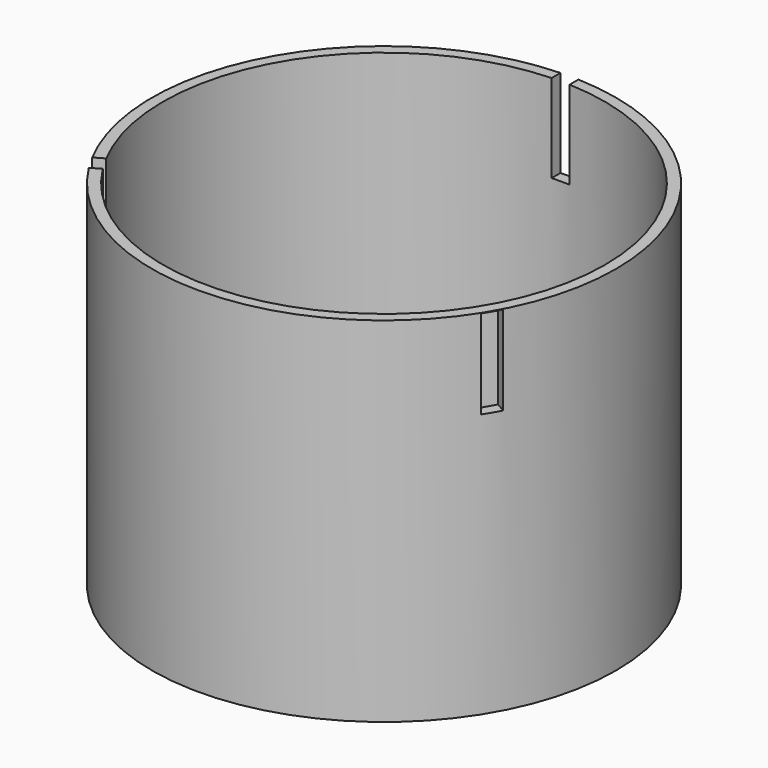
from build123d import *

# Parameters (mm, degrees)
F0_R           = 33.3375
F1_DEPTH       = 50.8
F2_T           = -1.5875
F6_W           = 2.5429241359
F6_H           = 13.1887868047
F7_DEPTH       = 12.7
F10_W          = 2.6744855568
F10_H          = 12.775093317
F11_DEPTH      = 2.794
F11_DEPTH_BACK = 2.413
F13_W          = 2.5820170995
F13_H          = 12.7615630627
F14_DEPTH      = 5.0546
F14_DEPTH_BACK = 4.7244
F15_W          = 7.62
F15_H          = 31.75
F15_R          = 1.397
F16_DEPTH      = 9.906


# Not quite as in the source:
# - a feature names something its author has since deleted; it is built from what else it names


with BuildPart() as f1:
    # F0 (on Top) → F1 (new body)
    with BuildSketch(Plane.XY):
        Circle(F0_R)
    extrude(amount=F1_DEPTH)

    # F2
    f2_openings = [f1.faces().sort_by_distance(p)[0] for p in [
        (0, 0, 50.8),
    ]]
    offset(amount=F2_T, openings=f2_openings)

    # F6 (on offset) → F7 (cut)
    with BuildSketch(Plane(origin=(-28.8711218987, -16.66875, 0), x_dir=(0.5, -0.8660254038, 0), z_dir=(-0.8660254038, -0.5, 0))):
        with Locations((0, 44.4019660354)):
            Rectangle(F6_W, F6_H)
    extrude(amount=-F7_DEPTH, mode=Mode.SUBTRACT)

    # F10 (on offset) → F11 (cut, two sides)
    with BuildSketch(Plane(origin=(28.8161292855, -16.637, 0), x_dir=(0.5, 0.8660254038, 0), z_dir=(0.8660254038, -0.5, 0))) as f11_sk:
        with Locations((0, 44.3391613662)):
            Rectangle(F10_W, F10_H)
    extrude(amount=-F11_DEPTH, mode=Mode.SUBTRACT)
    extrude(f11_sk.sketch, amount=F11_DEPTH_BACK, mode=Mode.SUBTRACT)

    # F13 (on offset) → F14 (cut, two sides)
    with BuildSketch(Plane.XZ.offset(-33.81375)) as f14_sk:
        with Locations((0, 44.5175170898)):
            Rectangle(F13_W, F13_H)
    extrude(amount=-F14_DEPTH, mode=Mode.SUBTRACT)
    extrude(f14_sk.sketch, amount=F14_DEPTH_BACK, mode=Mode.SUBTRACT)

    # F15 (on Top) → F16 (cut)
    with BuildSketch(Plane.XY):
        with Locations((-8.89, 0)):
            Rectangle(F15_W, F15_H)
        with Locations((-21.6036192909, 4.2545016563)):
            Circle(F15_R)
        with Locations((3.7963807091, 4.2545016563)):
            Circle(F15_R)
        with Locations((-8.9036192909, 22.3520016563)):
            Circle(F15_R)
    extrude(amount=F16_DEPTH, mode=Mode.SUBTRACT)


solid = f1.part
